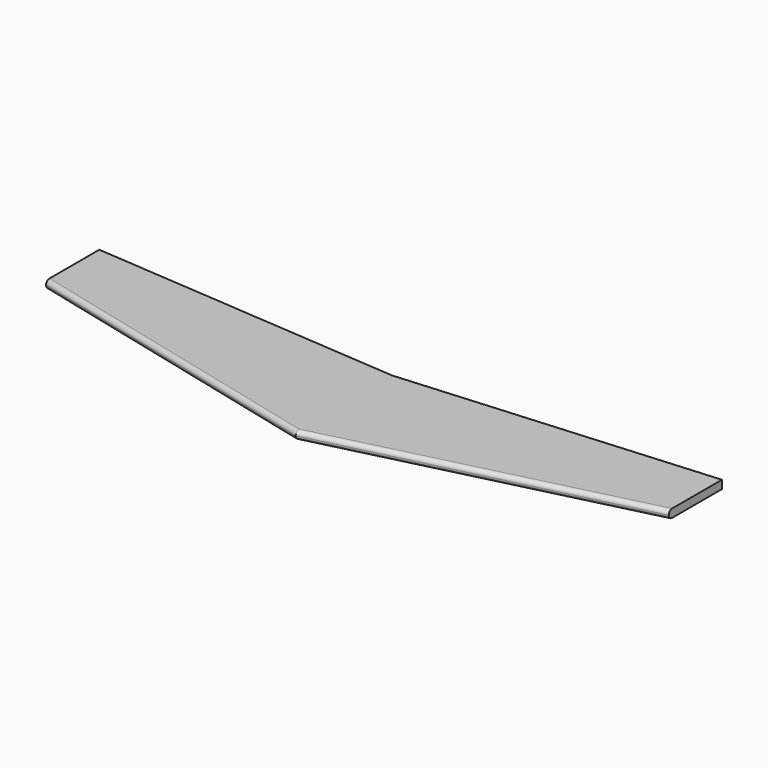
from build123d import *

# Parameters (mm, degrees)
F1_DEPTH = 5
F2_R     = 2.5
F3_R     = 2.49999
F7_ANGLE = 180


# Not quite as in the source:
# - a fillet or chamfer is up to 0.001 mm smaller than in the source, because OpenCascade refuses the exact size


with BuildPart() as f1:
    # F0 (on Top) → F1 (new body)
    with BuildSketch(Plane.XY):
        Polygon((0, 72.5676417351), (0, 0), (187.6123100519, -13.9679014683), (187.6123100519, 26.09346807), align=None)
    extrude(amount=F1_DEPTH)

    # F2
    f2_edges = [f1.edges().sort_by_distance(p)[0] for p in [
        (93.806155, 49.330555, 5),
    ]]
    fillet(f2_edges, radius=F2_R)

    # F3 (radius 2.5 in the source; OpenCascade refuses exactly that, so slightly less here)
    f3_edges = [f1.edges().sort_by_distance(p)[0] for p in [
        (93.806155, 49.330555, 0),
    ]]
    fillet(f3_edges, radius=F3_R)


with BuildPart() as f4_1:
    # F4: instance of F1
    add(f1.part.mirror(Plane.YZ))


with BuildPart() as f1_1:
    add(f1.part)

    add(f4_1.part)  # F5 merges F4_1
    # F5: F1 across plane
    add(f1.part.mirror(Plane.YZ))


with BuildPart() as f1_2:
    # F7: moved
    add(f1_1.part.rotate(Axis((0, 0, 62.2569620609), (0, 0, 1)), F7_ANGLE))


solid = f1_2.part
